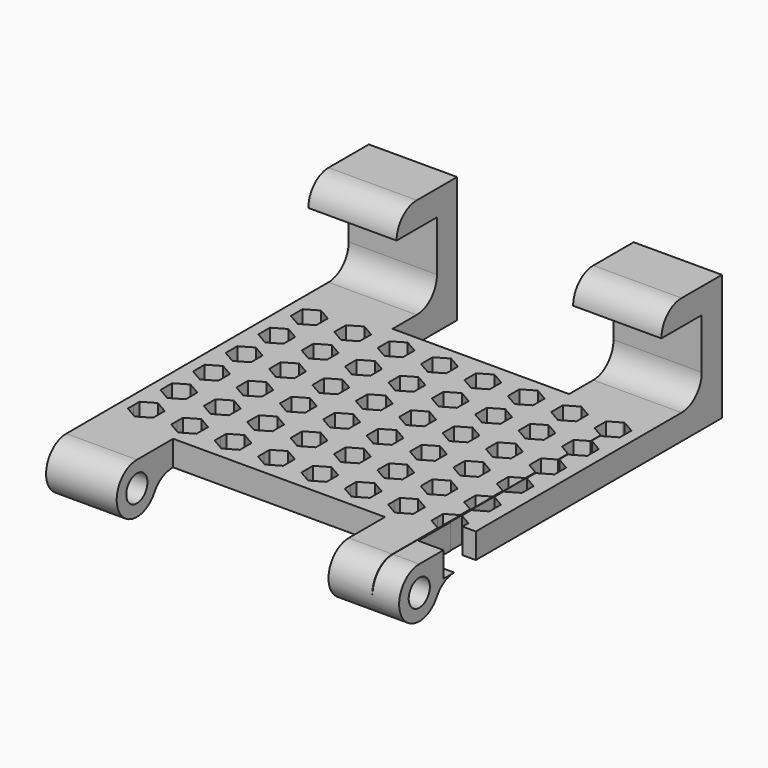
from build123d import *

# Parameters (mm, degrees)
F0_R          = 2.625
F1_DEPTH      = 70
F2_W          = 35
F2_H          = 25
F3_DEPTH      = 16
F5_W          = 42
F5_H          = 10
F6_DEPTH      = 9
F6_DEPTH_BACK = 5.001
F7_R          = 5
F8_R          = 4.99999
F9_W          = 0.0662033292
F9_H          = 7.9997260653
F10_DEPTH     = 15


# Not quite as in the source:
# - a fillet or chamfer is up to 0.001 mm smaller than in the source, because OpenCascade refuses the exact size


with BuildPart() as f1:
    # F0 (on Right) → F1 (new body)
    with BuildSketch(Plane.YZ):
        with BuildLine():
            Line((-5, 5), (-20.3439258039, 5))
            Line((-20.3439258039, 5), (-75, 5))
            ThreePointArc((-75, 5), (-79.3301270189, -2.5), (-70.6698729811, -2.5))
            ThreePointArc((-70.6698729811, -2.5), (-68.8397459622, -0.6698729811), (-66.3397459622, 0))
            Line((-66.3397459622, 0), (0, 0))
            Line((0, 0), (0, 5))
            Line((0, 5), (0, 25))
            Line((0, 25), (-15, 25))
            Line((-15, 25), (-15, 20))
            Line((-15, 20), (-5, 20))
            Line((-5, 20), (-5, 5))
        make_face()
        with Locations((-75, 0)):
            Circle(F0_R, mode=Mode.SUBTRACT)
    extrude(amount=F1_DEPTH)

    # F2 (on Front) → F3 (cut)
    with BuildSketch(Plane.XZ):
        with Locations((35, 12.5)):
            Rectangle(F2_W, F2_H)
    extrude(amount=F3_DEPTH, mode=Mode.SUBTRACT)

    # F5 (on offset) → F6 (cut, two sides)
    with BuildSketch(Plane.XZ.offset(75)) as f6_sk:
        with Locations((35, 0)):
            Rectangle(F5_W, F5_H)
    extrude(amount=-F6_DEPTH, mode=Mode.SUBTRACT)
    extrude(f6_sk.sketch, amount=F6_DEPTH_BACK, mode=Mode.SUBTRACT)

    # F7
    f7_edges = [f1.edges().sort_by_distance(p)[0] for p in [
        (8.75, -5, 5),
        (61.25, -5, 5),
    ]]
    fillet(f7_edges, radius=F7_R)

    # F8 (radius 5 in the source; OpenCascade refuses exactly that, so slightly less here)
    f8_edges = [f1.edges().sort_by_distance(p)[0] for p in [
        (8.75, -15, 25),
        (61.25, -15, 25),
    ]]
    fillet(f8_edges, radius=F8_R)

    # F9 (on Top) → F10 (cut)
    with BuildSketch(Plane.XY):
        Polygon((5.0001346615, -18.1132486541), (2.5000673308, -19.5565077067), (2.4999326692, -22.4432590527), (4.9998653385, -23.8867513459), (7.4999326692, -22.4434922933), (7.5000673308, -19.5567409473), align=None)
        Polygon((2.1690506849, -59.555138033), (2.1689832848, -61), (7.047863093, -61), (7.1689832957, -61), (7.1690506849, -59.5553712736), (4.6691180157, -58.1118789804), align=None)
        Polygon((7.047863093, -61), (2.1689832848, -61), (2.1689160234, -62.441889379), (4.6688486927, -63.8853816723), (7.1689160234, -62.4421226196), (7.1689832957, -61), align=None)
        Polygon((62.3690506849, -59.555138033), (62.3689832848, -61), (64.6689833542, -61), (64.6689833542, -58.2274143335), align=None)
        Polygon((64.6689833542, -61), (62.3689832848, -61), (62.3689160234, -62.441889379), (64.6689833542, -63.7699769338), align=None)
        Polygon((53.7690506849, -59.555138033), (53.7689832848, -61), (58.7689832957, -61), (58.7690506849, -59.5553712736), (56.2691180157, -58.1118789804), align=None)
        Polygon((58.7689832957, -61), (53.7689832848, -61), (53.7689160234, -62.441889379), (56.2688486927, -63.8853816723), (58.7689160234, -62.4421226196), align=None)
        Polygon((45.1690506849, -59.555138033), (45.1689832848, -61), (50.047863093, -61), (50.1689832957, -61), (50.1690506849, -59.5553712736), (47.6691180157, -58.1118789804), align=None)
        Polygon((50.047863093, -61), (45.1689832848, -61), (45.1689160234, -62.441889379), (47.6688486927, -63.8853816723), (50.1689160234, -62.4421226196), (50.1689832957, -61), align=None)
        Polygon((36.5690506849, -59.555138033), (36.5689832848, -61), (41.447863093, -61), (41.5689832957, -61), (41.5690506849, -59.5553712736), (39.0691180157, -58.1118789804), align=None)
        Polygon((41.447863093, -61), (36.5689832848, -61), (36.5689160234, -62.441889379), (39.0688486927, -63.8853816723), (41.5689160234, -62.4421226196), (41.5689832957, -61), align=None)
        Polygon((27.9690506849, -59.555138033), (27.9689832848, -61), (32.847863093, -61), (32.9689832957, -61), (32.9690506849, -59.5553712736), (30.4691180157, -58.1118789804), align=None)
        Polygon((32.847863093, -61), (27.9689832848, -61), (27.9689160234, -62.441889379), (30.4688486927, -63.8853816723), (32.9689160234, -62.4421226196), (32.9689832957, -61), align=None)
        Polygon((19.3690506849, -59.555138033), (19.3689832848, -61), (24.247863093, -61), (24.3689832957, -61), (24.3690506849, -59.5553712736), (21.8691180157, -58.1118789804), align=None)
        Polygon((24.247863093, -61), (19.3689832848, -61), (19.3689160234, -62.441889379), (21.8688486927, -63.8853816723), (24.3689160234, -62.4421226196), (24.3689832957, -61), align=None)
        Polygon((10.7690506849, -59.555138033), (10.7689832848, -61), (15.647863093, -61), (15.7689832957, -61), (15.7690506849, -59.5553712736), (13.2691180157, -58.1118789804), align=None)
        Polygon((15.647863093, -61), (10.7689832848, -61), (10.7689160234, -62.441889379), (13.2688486927, -63.8853816723), (15.7689160234, -62.4421226196), (15.7689832957, -61), align=None)
        Polygon((64.6689833542, -58.2274143335), (64.6689833542, -61), (64.7351866833, -61), (64.7351866833, -58.1891959412), align=None)
        Polygon((64.7351866833, -61), (64.6689833542, -61), (64.6689833542, -63.7699769338), (64.7351866833, -63.8082035615), align=None)
        Polygon((64.7351866833, -63.8082035615), (64.6689833542, -63.7699769338), (64.6689833542, -68.9997260653), (64.7351866833, -68.9997260653), align=None)
        Polygon((64.6689833542, -55.7320242409), (64.6689833542, -58.2274143335), (64.7351866833, -58.1891959412), (64.7351866833, -55.7702508686), align=None)
        with Locations((64.7020850188, -72.9995890979)):
            Rectangle(F9_W, F9_H)
        Polygon((62.4351193526, -54.4421633137), (64.6689833542, -55.7320242409), (64.6689833542, -50.2659066606), (62.4352540141, -51.5554119678), align=None)
        Polygon((64.6689833542, -50.2659066606), (64.6689833542, -55.7320242409), (64.7351866833, -55.7702508686), (64.7351866833, -50.2276882683), align=None)
        Polygon((64.7351866833, -50.2276882683), (64.7351866833, -55.7702508686), (64.8013900125, -55.8084774963), (64.8013900125, -50.1894698759), align=None)
        with Locations((64.7020850188, -80.9993151632)):
            Rectangle(F9_W, F9_H)
        Polygon((64.9337966708, -58.1492252423), (64.9337966708, -61), (65, -61), (65, -58.18745187), align=None)
        Polygon((64.7351866833, -47.7322981756), (64.7351866833, -50.2276882683), (64.8013900125, -50.1894698759), (64.8013900125, -47.7705248033), align=None)
        with Locations((64.7020850188, -88.9990412284)):
            Rectangle(F9_W, F9_H)
        Polygon((65, -58.18745187), (65, -61), (67.3689832957, -61), (67.3690506849, -59.5553712736), align=None)
        Polygon((67.3689832957, -61), (65, -61), (65, -63.8096695867), (67.3689160234, -62.4421226196), align=None)
        Polygon((64.9337966708, -55.8849307517), (64.9337966708, -58.1492252423), (65, -58.18745187), (65, -55.8481619138), (64.9350520218, -55.885655607), align=None)
        Polygon((62.5013226817, -46.4424372485), (64.7351866833, -47.7322981756), (64.7351866833, -42.2661805953), (62.5014573433, -43.5556859025), align=None)
        Polygon((64.7351866833, -42.2661805953), (64.7351866833, -47.7322981756), (64.8013900125, -47.7705248033), (64.8013900125, -42.227962203), align=None)
        with Locations((64.7020850188, -96.9987672937)):
            Rectangle(F9_W, F9_H)
        Polygon((71.8478709459, -61), (67.3689832957, -61), (67.3689160234, -62.4421226196), (65, -63.8096695867), (65, -68.9997260653), (71.7816676168, -68.9997260653), (73.2689833542, -68.9997260653), (73.2689833542, -61), align=None)
        Polygon((64.9337966708, -50.1130330912), (64.9337966708, -55.8849307517), (64.9350520218, -55.885655607), (65, -55.8481619138), (65, -50.149499177), (64.9353213449, -50.1121529151), align=None)
        Polygon((64.8013900125, -42.227962203), (64.8013900125, -47.7705248033), (64.8675933417, -47.808751431), (64.8675933417, -42.1897438107), align=None)
        with Locations((64.7682883479, -96.9987672937)):
            Rectangle(F9_W, F9_H)
        Polygon((65, -50.149499177), (65, -55.8481619138), (67.4351193526, -54.4423965543), (67.4352540141, -51.5556452084), align=None)
        Polygon((64.9337966708, -47.8469780587), (64.9337966708, -50.1130330912), (64.9353213449, -50.1121529151), (65, -50.149499177), (65, -47.8852046864), align=None)
        Polygon((64.8675933417, -92.998904261), (64.8013900125, -92.998904261), (64.8013900125, -100.9986303263), (71.5168543001, -100.9986303263), (73.2689833542, -100.9986303263), (73.2689833542, -92.998904261), (71.5830576293, -92.998904261), align=None)
        Polygon((64.8013900125, -39.7325721103), (64.8013900125, -42.227962203), (64.8675933417, -42.1897438107), (64.8675933417, -39.770798738), align=None)
        with Locations((73.3020850188, -64.9998630326)):
            Rectangle(F9_W, F9_H)
        Polygon((64.9337966708, -42.1515254183), (64.9337966708, -47.8469780587), (65, -47.8852046864), (65, -42.113307026), align=None)
        Polygon((62.5675260109, -38.4427111832), (64.8013900125, -39.7325721103), (64.8013900125, -34.2664545301), (62.5676606724, -35.5559598372), align=None)
        Polygon((64.8013900125, -34.2664545301), (64.8013900125, -39.7325721103), (64.8675933417, -39.770798738), (64.8675933417, -34.2282361377), align=None)
        with Locations((73.3682883479, -64.9998630326)):
            Rectangle(F9_W, F9_H)
        Polygon((65, -42.113307026), (65, -47.8852046864), (65.001255351, -47.8859295417), (67.5013226817, -46.4426704891), (67.5014573433, -43.5559191431), (65.001524674, -42.1124268498), align=None)
        Polygon((64.9337966708, -39.8090253657), (64.9337966708, -42.1515254183), (65, -42.113307026), (65, -39.8472519935), align=None)
        Polygon((64.8675933417, -34.2282361377), (64.8675933417, -39.770798738), (64.9337966708, -39.8090253657), (64.9337966708, -34.1900177454), align=None)
        with Locations((73.4344916771, -64.9998630326)):
            Rectangle(F9_W, F9_H)
        Polygon((64.9337966708, -34.1900177454), (64.9337966708, -39.8090253657), (65, -39.8472519935), (65, -34.151799353), align=None)
        with Locations((73.3020850188, -96.9987672937)):
            Rectangle(F9_W, F9_H)
        Polygon((64.8675933417, -31.7328460451), (64.8675933417, -34.2282361377), (64.9337966708, -34.1900177454), (64.9337966708, -31.7710726728), align=None)
        with Locations((73.5006950063, -64.9998630326)):
            Rectangle(F9_W, F9_H)
        Polygon((65, -34.151799353), (65, -39.8472519935), (65.0674586801, -39.8862034765), (67.5675260109, -38.4429444238), (67.5676606724, -35.5561930778), (65.0677280032, -34.1127007846), align=None)
        Polygon((64.9337966708, -31.7710726728), (64.9337966708, -34.1900177454), (65, -34.151799353), (65, -31.8092993005), align=None)
        with Locations((73.3682883479, -96.9987672937)):
            Rectangle(F9_W, F9_H)
        Polygon((62.6337293401, -30.4429851179), (64.8675933417, -31.7328460451), (64.8675933417, -26.2667284648), (62.6338640016, -27.556233772), align=None)
        Polygon((64.8675933417, -26.2667284648), (64.8675933417, -31.7328460451), (64.9337966708, -31.7710726728), (64.9337966708, -26.2285100725), align=None)
        with Locations((73.5668983354, -64.9998630326)):
            Rectangle(F9_W, F9_H)
        Polygon((64.9337966708, -26.2285100725), (64.9337966708, -31.7710726728), (65, -31.8092993005), (65, -26.1902916801), align=None)
        Polygon((73.4675933417, -92.998904261), (73.4013900125, -92.998904261), (73.4013900125, -100.9986303263), (80.1168543001, -100.9986303263), (81.8689833542, -100.9986303263), (81.8689833542, -92.998904261), (80.1830576293, -92.998904261), align=None)
        Polygon((80.4478709459, -61), (73.6, -61), (73.6, -68.9997260653), (80.3816676168, -68.9997260653), (81.8689833542, -68.9997260653), (81.8689833542, -61), align=None)
        Polygon((65, -26.1902916801), (65, -31.8092993005), (65.1336620093, -31.8864774112), (67.6337293401, -30.4432183585), (67.6338640016, -27.5564670126), (65.1339313324, -26.1129747193), align=None)
        Polygon((64.9337966708, -23.7331199798), (64.9337966708, -26.2285100725), (65, -26.1902916801), (65, -23.7713466075), align=None)
        Polygon((62.6999326692, -22.4432590527), (64.9337966708, -23.7331199798), (64.9337966708, -18.2670023996), (62.7000673308, -19.5565077067), align=None)
        Polygon((64.9337966708, -18.2670023996), (64.9337966708, -23.7331199798), (65, -23.7713466075), (65, -18.2287840072), align=None)
        with Locations((81.9020850188, -96.9987672937)):
            Rectangle(F9_W, F9_H)
        with Locations((81.9020850188, -64.9998630326)):
            Rectangle(F9_W, F9_H)
        Polygon((65, -18.2287840072), (65, -23.7713466075), (65.1998653385, -23.8867513459), (67.6999326692, -22.4434922933), (67.7000673308, -19.5567409473), (65.2001346615, -18.1132486541), align=None)
        with Locations((81.9682883479, -96.9987672937)):
            Rectangle(F9_W, F9_H)
        with Locations((81.9682883479, -64.9998630326)):
            Rectangle(F9_W, F9_H)
        Polygon((82.0013900125, -92.998904261), (82.0013900125, -100.9986303263), (88.7168543001, -100.9986303263), (90.4689833542, -100.9986303263), (90.4689833542, -92.998904261), (88.7830576293, -92.998904261), (82.0675933417, -92.998904261), align=None)
        with Locations((82.0344916771, -64.9998630326)):
            Rectangle(F9_W, F9_H)
        with Locations((82.1006950063, -64.9998630326)):
            Rectangle(F9_W, F9_H)
        with Locations((90.5020850188, -96.9987672937)):
            Rectangle(F9_W, F9_H)
        with Locations((82.1668983354, -64.9998630326)):
            Rectangle(F9_W, F9_H)
        with Locations((90.5682883479, -96.9987672937)):
            Rectangle(F9_W, F9_H)
        Polygon((89.0478709459, -61), (82.2, -61), (82.2, -68.9997260653), (88.9816676168, -68.9997260653), (90.4689833542, -68.9997260653), (90.4689833542, -61), align=None)
        Polygon((90.6013900125, -92.998904261), (90.6013900125, -100.9986303263), (97.3168543001, -100.9986303263), (99.0689833542, -100.9986303263), (99.0689833542, -92.998904261), (97.3830576293, -92.998904261), (90.6675933417, -92.998904261), align=None)
        with Locations((90.5020850188, -64.9998630326)):
            Rectangle(F9_W, F9_H)
        with Locations((99.1020850188, -96.9987672937)):
            Rectangle(F9_W, F9_H)
        with Locations((90.5682883479, -64.9998630326)):
            Rectangle(F9_W, F9_H)
        with Locations((99.1682883479, -96.9987672937)):
            Rectangle(F9_W, F9_H)
        with Locations((90.6344916771, -64.9998630326)):
            Rectangle(F9_W, F9_H)
        Polygon((99.2013900125, -92.998904261), (99.2013900125, -100.9986303263), (105.9168543001, -100.9986303263), (107.6689833542, -100.9986303263), (107.6689833542, -92.998904261), (105.9830576293, -92.998904261), (99.2675933417, -92.998904261), align=None)
        with Locations((90.7006950063, -64.9998630326)):
            Rectangle(F9_W, F9_H)
        with Locations((90.7668983354, -64.9998630326)):
            Rectangle(F9_W, F9_H)
        with Locations((107.7020850188, -96.9987672937)):
            Rectangle(F9_W, F9_H)
        with Locations((99.1020850188, -64.9998630326)):
            Rectangle(F9_W, F9_H)
        Polygon((97.5816676168, -68.9997260653), (99.0689833542, -68.9997260653), (99.0689833542, -61), (97.6478709459, -61), (90.8, -61), (90.8, -68.9997260653), align=None)
        with Locations((99.1682883479, -64.9998630326)):
            Rectangle(F9_W, F9_H)
        with Locations((107.7682883479, -96.9987672937)):
            Rectangle(F9_W, F9_H)
        with Locations((99.2344916771, -64.9998630326)):
            Rectangle(F9_W, F9_H)
        Polygon((107.8013900125, -92.998904261), (107.8013900125, -100.9986303263), (114.5168543001, -100.9986303263), (116.2689833542, -100.9986303263), (116.2689833542, -92.998904261), (114.5830576293, -92.998904261), (107.8675933417, -92.998904261), align=None)
        with Locations((99.3006950063, -64.9998630326)):
            Rectangle(F9_W, F9_H)
        with Locations((99.3668983354, -64.9998630326)):
            Rectangle(F9_W, F9_H)
        with Locations((116.3020850188, -96.9987672937)):
            Rectangle(F9_W, F9_H)
        with Locations((107.7020850188, -64.9998630326)):
            Rectangle(F9_W, F9_H)
        Polygon((106.1816676168, -68.9997260653), (107.6689833542, -68.9997260653), (107.6689833542, -61), (106.2478709459, -61), (99.4, -61), (99.4, -68.9997260653), align=None)
        with Locations((107.7682883479, -64.9998630326)):
            Rectangle(F9_W, F9_H)
        with Locations((116.3682883479, -96.9987672937)):
            Rectangle(F9_W, F9_H)
        with Locations((107.8344916771, -64.9998630326)):
            Rectangle(F9_W, F9_H)
        Polygon((116.4013900125, -92.998904261), (116.4013900125, -100.9986303263), (123.1168543001, -100.9986303263), (124.8689833542, -100.9986303263), (124.8689833542, -92.998904261), (123.1830576293, -92.998904261), (116.4675933417, -92.998904261), align=None)
        with Locations((107.9006950063, -64.9998630326)):
            Rectangle(F9_W, F9_H)
        with Locations((107.9668983354, -64.9998630326)):
            Rectangle(F9_W, F9_H)
        with Locations((124.9020850188, -96.9987672937)):
            Rectangle(F9_W, F9_H)
        with Locations((116.3020850188, -64.9998630326)):
            Rectangle(F9_W, F9_H)
        Polygon((114.7816676168, -68.9997260653), (116.2689833542, -68.9997260653), (116.2689833542, -61), (114.8478709459, -61), (108, -61), (108, -68.9997260653), align=None)
        with Locations((116.3682883479, -64.9998630326)):
            Rectangle(F9_W, F9_H)
        with Locations((124.9682883479, -96.9987672937)):
            Rectangle(F9_W, F9_H)
        with Locations((116.4344916771, -64.9998630326)):
            Rectangle(F9_W, F9_H)
        with Locations((124.9682883479, -88.9990412284)):
            Rectangle(F9_W, F9_H)
        with Locations((116.5006950063, -64.9998630326)):
            Rectangle(F9_W, F9_H)
        with Locations((125.0344916771, -88.9990412284)):
            Rectangle(F9_W, F9_H)
        with Locations((116.5668983354, -64.9998630326)):
            Rectangle(F9_W, F9_H)
        with Locations((125.0344916771, -80.9993151632)):
            Rectangle(F9_W, F9_H)
        with Locations((124.9020850188, -64.9998630326)):
            Rectangle(F9_W, F9_H)
        Polygon((123.3816676168, -68.9997260653), (124.8689833542, -68.9997260653), (124.8689833542, -61), (123.4478709459, -61), (116.6, -61), (116.6, -68.9997260653), align=None)
        with Locations((125.1006950063, -80.9993151632)):
            Rectangle(F9_W, F9_H)
        with Locations((124.9682883479, -64.9998630326)):
            Rectangle(F9_W, F9_H)
        with Locations((125.1006950063, -72.9995890979)):
            Rectangle(F9_W, F9_H)
        with Locations((125.0344916771, -64.9998630326)):
            Rectangle(F9_W, F9_H)
        with Locations((125.1668983354, -72.9995890979)):
            Rectangle(F9_W, F9_H)
        with Locations((125.1006950063, -64.9998630326)):
            Rectangle(F9_W, F9_H)
        with Locations((125.1668983354, -64.9998630326)):
            Rectangle(F9_W, F9_H)
        Polygon((2.4338640016, -27.556233772), (2.4337293401, -30.4429851179), (4.9336620093, -31.8864774112), (7.4337293401, -30.4432183585), (7.4338640016, -27.5564670126), (4.9339313324, -26.1129747193), align=None)
        Polygon((2.3676606724, -35.5559598372), (2.3675260109, -38.4427111832), (4.8674586801, -39.8862034765), (7.3675260109, -38.4429444238), (7.3676606724, -35.5561930778), (4.8677280032, -34.1127007846), align=None)
        Polygon((2.3014573433, -43.5556859025), (2.3013226817, -46.4424372485), (4.801255351, -47.8859295417), (7.3013226817, -46.4426704891), (7.3014573433, -43.5559191431), (4.801524674, -42.1124268498), align=None)
        Polygon((2.2352540141, -51.5554119678), (2.2351193526, -54.4421633137), (4.7350520218, -55.885655607), (7.2351193526, -54.4423965543), (7.2352540141, -51.5556452084), (4.7353213449, -50.1121529151), align=None)
        Polygon((11.1000673308, -19.5565077067), (11.0999326692, -22.4432590527), (13.5998653385, -23.8867513459), (16.0999326692, -22.4434922933), (16.1000673308, -19.5567409473), (13.6001346615, -18.1132486541), align=None)
        Polygon((11.0338640016, -27.556233772), (11.0337293401, -30.4429851179), (13.5336620093, -31.8864774112), (16.0337293401, -30.4432183585), (16.0338640016, -27.5564670126), (13.5339313324, -26.1129747193), align=None)
        Polygon((10.9676606724, -35.5559598372), (10.9675260109, -38.4427111832), (13.4674586801, -39.8862034765), (15.9675260109, -38.4429444238), (15.9676606724, -35.5561930778), (13.4677280032, -34.1127007846), align=None)
        Polygon((10.9014573433, -43.5556859025), (10.9013226817, -46.4424372485), (13.401255351, -47.8859295417), (15.9013226817, -46.4426704891), (15.9014573433, -43.5559191431), (13.401524674, -42.1124268498), align=None)
        Polygon((10.8352540141, -51.5554119678), (10.8351193526, -54.4421633137), (13.3350520218, -55.885655607), (15.8351193526, -54.4423965543), (15.8352540141, -51.5556452084), (13.3353213449, -50.1121529151), align=None)
        Polygon((19.7000673308, -19.5565077067), (19.6999326692, -22.4432590527), (22.1998653385, -23.8867513459), (24.6999326692, -22.4434922933), (24.7000673308, -19.5567409473), (22.2001346615, -18.1132486541), align=None)
        Polygon((19.6338640016, -27.556233772), (19.6337293401, -30.4429851179), (22.1336620093, -31.8864774112), (24.6337293401, -30.4432183585), (24.6338640016, -27.5564670126), (22.1339313324, -26.1129747193), align=None)
        Polygon((19.5676606724, -35.5559598372), (19.5675260109, -38.4427111832), (22.0674586801, -39.8862034765), (24.5675260109, -38.4429444238), (24.5676606724, -35.5561930778), (22.0677280032, -34.1127007846), align=None)
        Polygon((19.5014573433, -43.5556859025), (19.5013226817, -46.4424372485), (22.001255351, -47.8859295417), (24.5013226817, -46.4426704891), (24.5014573433, -43.5559191431), (22.001524674, -42.1124268498), align=None)
        Polygon((19.4352540141, -51.5554119678), (19.4351193526, -54.4421633137), (21.9350520218, -55.885655607), (24.4351193526, -54.4423965543), (24.4352540141, -51.5556452084), (21.9353213449, -50.1121529151), align=None)
        Polygon((28.3000673308, -19.5565077067), (28.2999326692, -22.4432590527), (30.7998653385, -23.8867513459), (33.2999326692, -22.4434922933), (33.3000673308, -19.5567409473), (30.8001346615, -18.1132486541), align=None)
        Polygon((28.2338640016, -27.556233772), (28.2337293401, -30.4429851179), (30.7336620093, -31.8864774112), (33.2337293401, -30.4432183585), (33.2338640016, -27.5564670126), (30.7339313324, -26.1129747193), align=None)
        Polygon((28.1676606724, -35.5559598372), (28.1675260109, -38.4427111832), (30.6674586801, -39.8862034765), (33.1675260109, -38.4429444238), (33.1676606724, -35.5561930778), (30.6677280032, -34.1127007846), align=None)
        Polygon((28.1014573433, -43.5556859025), (28.1013226817, -46.4424372485), (30.601255351, -47.8859295417), (33.1013226817, -46.4426704891), (33.1014573433, -43.5559191431), (30.601524674, -42.1124268498), align=None)
        Polygon((28.0352540141, -51.5554119678), (28.0351193526, -54.4421633137), (30.5350520218, -55.885655607), (33.0351193526, -54.4423965543), (33.0352540141, -51.5556452084), (30.5353213449, -50.1121529151), align=None)
        Polygon((36.9000673308, -19.5565077067), (36.8999326692, -22.4432590527), (39.3998653385, -23.8867513459), (41.8999326692, -22.4434922933), (41.9000673308, -19.5567409473), (39.4001346615, -18.1132486541), align=None)
        Polygon((36.8338640016, -27.556233772), (36.8337293401, -30.4429851179), (39.3336620093, -31.8864774112), (41.8337293401, -30.4432183585), (41.8338640016, -27.5564670126), (39.3339313324, -26.1129747193), align=None)
        Polygon((36.7676606724, -35.5559598372), (36.7675260109, -38.4427111832), (39.2674586801, -39.8862034765), (41.7675260109, -38.4429444238), (41.7676606724, -35.5561930778), (39.2677280032, -34.1127007846), align=None)
        Polygon((36.7014573433, -43.5556859025), (36.7013226817, -46.4424372485), (39.201255351, -47.8859295417), (41.7013226817, -46.4426704891), (41.7014573433, -43.5559191431), (39.201524674, -42.1124268498), align=None)
        Polygon((36.6352540141, -51.5554119678), (36.6351193526, -54.4421633137), (39.1350520218, -55.885655607), (41.6351193526, -54.4423965543), (41.6352540141, -51.5556452084), (39.1353213449, -50.1121529151), align=None)
        Polygon((45.5000673308, -19.5565077067), (45.4999326692, -22.4432590527), (47.9998653385, -23.8867513459), (50.4999326692, -22.4434922933), (50.5000673308, -19.5567409473), (48.0001346615, -18.1132486541), align=None)
        Polygon((45.4338640016, -27.556233772), (45.4337293401, -30.4429851179), (47.9336620093, -31.8864774112), (50.4337293401, -30.4432183585), (50.4338640016, -27.5564670126), (47.9339313324, -26.1129747193), align=None)
        Polygon((45.3676606724, -35.5559598372), (45.3675260109, -38.4427111832), (47.8674586801, -39.8862034765), (50.3675260109, -38.4429444238), (50.3676606724, -35.5561930778), (47.8677280032, -34.1127007846), align=None)
        Polygon((45.3014573433, -43.5556859025), (45.3013226817, -46.4424372485), (47.801255351, -47.8859295417), (50.3013226817, -46.4426704891), (50.3014573433, -43.5559191431), (47.801524674, -42.1124268498), align=None)
        Polygon((45.2352540141, -51.5554119678), (45.2351193526, -54.4421633137), (47.7350520218, -55.885655607), (50.2351193526, -54.4423965543), (50.2352540141, -51.5556452084), (47.7353213449, -50.1121529151), align=None)
        Polygon((54.1000673308, -19.5565077067), (54.0999326692, -22.4432590527), (56.5998653385, -23.8867513459), (59.0999326692, -22.4434922933), (59.1000673308, -19.5567409473), (56.6001346615, -18.1132486541), align=None)
        Polygon((54.0338640016, -27.556233772), (54.0337293401, -30.4429851179), (56.5336620093, -31.8864774112), (59.0337293401, -30.4432183585), (59.0338640016, -27.5564670126), (56.5339313324, -26.1129747193), align=None)
        Polygon((53.9676606724, -35.5559598372), (53.9675260109, -38.4427111832), (56.4674586801, -39.8862034765), (58.9675260109, -38.4429444238), (58.9676606724, -35.5561930778), (56.4677280032, -34.1127007846), align=None)
        Polygon((53.9014573433, -43.5556859025), (53.9013226817, -46.4424372485), (56.401255351, -47.8859295417), (58.9013226817, -46.4426704891), (58.9014573433, -43.5559191431), (56.401524674, -42.1124268498), align=None)
        Polygon((53.8352540141, -51.5554119678), (53.8351193526, -54.4421633137), (56.3350520218, -55.885655607), (58.8351193526, -54.4423965543), (58.8352540141, -51.5556452084), (56.3353213449, -50.1121529151), align=None)
    extrude(amount=F10_DEPTH, mode=Mode.SUBTRACT)


solid = f1.part
